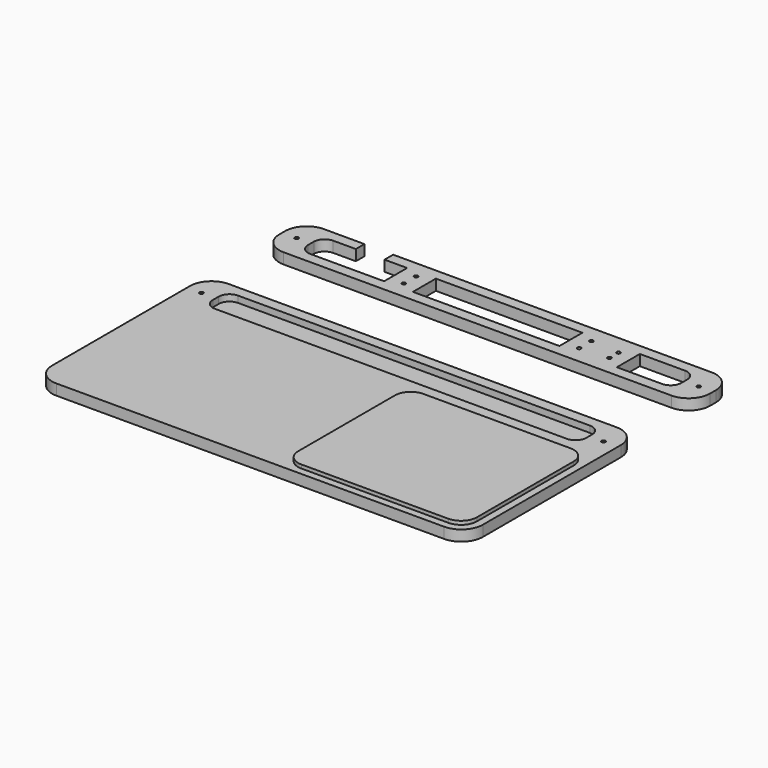
from build123d import *

# Parameters (mm, degrees)
F0_R     = 3.302
F0_W     = 259.2
F0_H     = 50.8
F1_DEPTH = 19.05
F2_DEPTH = 19.05
F3_DEPTH = 7.62
F4_DEPTH = 25.4


# Not quite as in the source:
# - a feature names something its author has since deleted; it is built from what else it names


with BuildPart() as f1:
    # F0 (on Top) → F1 (new body)
    with BuildSketch(Plane.XY):
        with BuildLine():
            ThreePointArc((-381, 350.0549432278), (-369.8407683632, 323.1141748646), (-342.9, 311.9549432278))
            Line((-342.9, 311.9549432278), (342.9, 311.9549432278))
            ThreePointArc((342.9, 311.9549432278), (369.8407683632, 323.1141748646), (381, 350.0549432278))
            Line((381, 350.0549432278), (381, 362.7549432278))
            ThreePointArc((381, 362.7549432278), (369.8407683632, 389.695711591), (342.9, 400.8549432278))
            Line((342.9, 400.8549432278), (-220.375, 400.8549432278))
            Line((-220.375, 400.8549432278), (-220.375, 381.8049432278))
            Line((-220.375, 381.8049432278), (-180.4, 381.8049432278))
            Line((-180.4, 381.8049432278), (-180.4, 331.0049432278))
            Line((-180.4, 331.0049432278), (-311.15, 331.0049432278))
            ThreePointArc((-311.15, 331.0049432278), (-324.6203841816, 336.5845590462), (-330.2, 350.0549432278))
            Line((-330.2, 350.0549432278), (-330.2, 362.7549432278))
            ThreePointArc((-330.2, 362.7549432278), (-324.6203841816, 376.2253274094), (-311.15, 381.8049432278))
            Line((-311.15, 381.8049432278), (-271.175, 381.8049432278))
            Line((-271.175, 381.8049432278), (-271.175, 400.8549432278))
            Line((-271.175, 400.8549432278), (-342.9, 400.8549432278))
            ThreePointArc((-342.9, 400.8549432278), (-369.8407683632, 389.695711591), (-381, 362.7549432278))
            Line((-381, 362.7549432278), (-381, 350.0549432278))
        make_face()
        with Locations((-355.6, 356.4049432278)):
            Circle(F0_R, mode=Mode.SUBTRACT)
        with BuildLine():
            ThreePointArc((-155, 339.6030464278), (-158.302, 342.9050464278), (-155, 346.2070464278))
            ThreePointArc((-155, 346.2070464278), (-152.6651334085, 345.2399130192), (-151.698, 342.9050464278))
            ThreePointArc((-151.698, 342.9050464278), (-152.6651334085, 340.5701798363), (-155, 339.6030464278))
        make_face(mode=Mode.SUBTRACT)
        with BuildLine():
            ThreePointArc((-155, 366.6030432278), (-158.302, 369.9050432278), (-155, 373.2070432278))
            ThreePointArc((-155, 373.2070432278), (-152.6651334085, 372.2399098192), (-151.698, 369.9050432278))
            ThreePointArc((-151.698, 369.9050432278), (-152.6651334085, 367.5701766363), (-155, 366.6030432278))
        make_face(mode=Mode.SUBTRACT)
        with Locations((0, 356.4049432278)):
            Rectangle(F0_W, F0_H, mode=Mode.SUBTRACT)
        with Locations((155, 342.9050464278)):
            Circle(F0_R, mode=Mode.SUBTRACT)
        with Locations((155, 369.9050432278)):
            Circle(F0_R, mode=Mode.SUBTRACT)
        with Locations((205.8, 346.4049378278)):
            Circle(F0_R, mode=Mode.SUBTRACT)
        with Locations((205.8, 366.4049486278)):
            Circle(F0_R, mode=Mode.SUBTRACT)
        with BuildLine():
            Line((231.2, 331.0049432278), (231.2, 381.8049432278))
            Line((231.2, 381.8049432278), (311.15, 381.8049432278))
            ThreePointArc((311.15, 381.8049432278), (324.6203841816, 376.2253274094), (330.2, 362.7549432278))
            Line((330.2, 362.7549432278), (330.2, 350.0549432278))
            ThreePointArc((330.2, 350.0549432278), (324.6203841816, 336.5845590462), (311.15, 331.0049432278))
            Line((311.15, 331.0049432278), (231.2, 331.0049432278))
        make_face(mode=Mode.SUBTRACT)
        with Locations((355.6, 356.4049432278)):
            Circle(F0_R, mode=Mode.SUBTRACT)
    extrude(amount=F1_DEPTH)


with BuildPart() as f2:
    # F0 (on Top) → F2 (new body)
    with BuildSketch(Plane.XY):
        with BuildLine():
            Line((-342.9, -190.5), (342.9, -190.5))
            ThreePointArc((342.9, -190.5), (369.8407683632, -179.3407683632), (381, -152.4))
            Line((381, -152.4), (381, 152.4))
            ThreePointArc((381, 152.4), (369.8407683632, 179.3407683632), (342.9, 190.5))
            Line((342.9, 190.5), (-342.9, 190.5))
            ThreePointArc((-342.9, 190.5), (-369.8407683632, 179.3407683632), (-381, 152.4))
            Line((-381, 152.4), (-381, -152.4))
            ThreePointArc((-381, -152.4), (-369.8407683632, -179.3407683632), (-342.9, -190.5))
        make_face()
        with BuildLine():
            ThreePointArc((368.3, -149.8), (360.0989898732, -169.5989898732), (340.3, -177.8))
            Line((340.3, -177.8), (80.07, -177.8))
            ThreePointArc((80.07, -177.8), (60.2710101268, -169.5989898732), (52.07, -149.8))
            Line((52.07, -149.8), (52.07, 64.2))
            ThreePointArc((52.07, 64.2), (60.2710101268, 83.9989898732), (80.07, 92.2))
            Line((80.07, 92.2), (340.3, 92.2))
            ThreePointArc((340.3, 92.2), (360.0989898732, 83.9989898732), (368.3, 64.2))
            Line((368.3, 64.2), (368.3, -149.8))
        make_face(mode=Mode.SUBTRACT)
        with Locations((-355.6, 146.05)):
            Circle(F0_R, mode=Mode.SUBTRACT)
        with BuildLine():
            ThreePointArc((-330.2, 152.4), (-324.6203841816, 165.8703841816), (-311.15, 171.45))
            Line((-311.15, 171.45), (311.15, 171.45))
            ThreePointArc((311.15, 171.45), (324.6203841816, 165.8703841816), (330.2, 152.4))
            Line((330.2, 152.4), (330.2, 139.7))
            ThreePointArc((330.2, 139.7), (324.6203841816, 126.2296158184), (311.15, 120.65))
            Line((311.15, 120.65), (-311.15, 120.65))
            ThreePointArc((-311.15, 120.65), (-324.6203841816, 126.2296158184), (-330.2, 139.7))
            Line((-330.2, 139.7), (-330.2, 152.4))
        make_face(mode=Mode.SUBTRACT)
        with Locations((355.6, 146.05)):
            Circle(F0_R, mode=Mode.SUBTRACT)
        with BuildLine():
            Line((80.07, -177.8), (340.3, -177.8))
            ThreePointArc((340.3, -177.8), (360.0989898732, -169.5989898732), (368.3, -149.8))
            Line((368.3, -149.8), (368.3, 64.2))
            ThreePointArc((368.3, 64.2), (360.0989898732, 83.9989898732), (340.3, 92.2))
            Line((340.3, 92.2), (80.07, 92.2))
            ThreePointArc((80.07, 92.2), (60.2710101268, 83.9989898732), (52.07, 64.2))
            Line((52.07, 64.2), (52.07, -149.8))
            ThreePointArc((52.07, -149.8), (60.2710101268, -169.5989898732), (80.07, -177.8))
        make_face()
    extrude(amount=F2_DEPTH)

    # F0 (on Top) → F3 (join)
    with BuildSketch(Plane.XY):
        with BuildLine():
            Line((311.15, 171.45), (-311.15, 171.45))
            ThreePointArc((-311.15, 171.45), (-324.6203841816, 165.8703841816), (-330.2, 152.4))
            Line((-330.2, 152.4), (-330.2, 139.7))
            ThreePointArc((-330.2, 139.7), (-324.6203841816, 126.2296158184), (-311.15, 120.65))
            Line((-311.15, 120.65), (311.15, 120.65))
            ThreePointArc((311.15, 120.65), (324.6203841816, 126.2296158184), (330.2, 139.7))
            Line((330.2, 139.7), (330.2, 152.4))
            ThreePointArc((330.2, 152.4), (324.6203841816, 165.8703841816), (311.15, 171.45))
        make_face()
    extrude(amount=F3_DEPTH)

    # F0 (on Top) → F4 (join)
    with BuildSketch(Plane.XY):
        with BuildLine():
            Line((80.07, -177.8), (340.3, -177.8))
            ThreePointArc((340.3, -177.8), (360.0989898732, -169.5989898732), (368.3, -149.8))
            Line((368.3, -149.8), (368.3, 64.2))
            ThreePointArc((368.3, 64.2), (360.0989898732, 83.9989898732), (340.3, 92.2))
            Line((340.3, 92.2), (80.07, 92.2))
            ThreePointArc((80.07, 92.2), (60.2710101268, 83.9989898732), (52.07, 64.2))
            Line((52.07, 64.2), (52.07, -149.8))
            ThreePointArc((52.07, -149.8), (60.2710101268, -169.5989898732), (80.07, -177.8))
        make_face()
    extrude(amount=F4_DEPTH)


solid = Compound([f1.part, f2.part])
